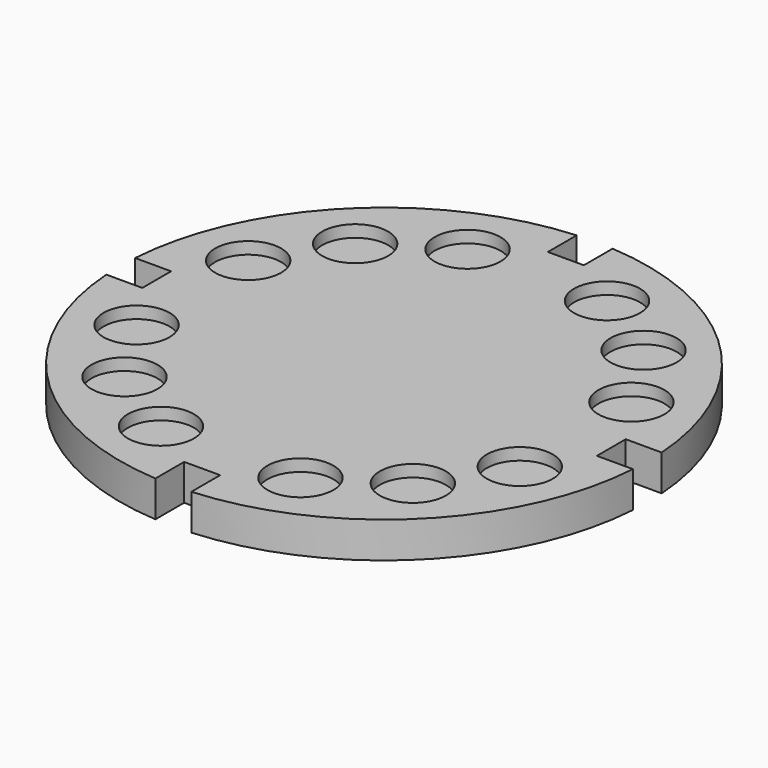
from build123d import *

# Parameters (mm, degrees)
F0_R            = 17.4625
F0_W            = 19.05
F0_H            = 6.35
F1_DEPTH        = 19.05
F2_DEPTH        = 6.35
F2_COPIES_COUNT = 4
F3_DEPTH        = 19.051
F3_COPIES_COUNT = 4


# Not quite as in the source:
# - a pattern or mirror of a feature is missing from the dataset's text; its kind, count and spacing are read off the source's solid


with BuildPart() as f1:
    # F0 (on Top) → F1 (new body)
    with BuildSketch(Plane.XY):
        with BuildLine():
            ThreePointArc((-9.525, 139.3749058296), (-95.3557746023, -102.0948884617), (139.7, 0))
            ThreePointArc((139.7, 0), (102.0948884617, 95.3557746023), (9.525, 139.3749058296))
            Line((9.525, 139.3749058296), (9.525, 120.3249058296))
            Line((9.525, 120.3249058296), (9.525, 113.9749058296))
            Line((9.525, 113.9749058296), (-9.525, 113.9749058296))
            Line((-9.525, 113.9749058296), (-9.525, 120.3249058296))
            Line((-9.525, 120.3249058296), (-9.525, 139.3749058296))
        make_face()
        with Locations((101.4398184138, 36.921074472)):
            Circle(F0_R, mode=Mode.SUBTRACT)
        with Locations((36.921074472, 101.4398184138)):
            Circle(F0_R, mode=Mode.SUBTRACT)
        with Locations((76.3321770291, 76.3321770291)):
            Circle(F0_R, mode=Mode.SUBTRACT)
        with BuildLine():
            Line((9.525, 120.3249058296), (9.525, 139.3749058296))
            ThreePointArc((9.525, 139.3749058296), (0, 139.7), (-9.525, 139.3749058296))
            Line((-9.525, 139.3749058296), (-9.525, 120.3249058296))
            Line((-9.525, 120.3249058296), (9.525, 120.3249058296))
        make_face()
        with Locations((36.921074472, 101.4398184138)):
            Circle(F0_R)
        with Locations((76.3321770291, 76.3321770291)):
            Circle(F0_R)
        with Locations((101.4398184138, 36.921074472)):
            Circle(F0_R)
        with Locations((0, 117.1499058296)):
            Rectangle(F0_W, F0_H)
    extrude(amount=-F1_DEPTH)

    # F0 (on Top) → F2 (cut)
    with BuildSketch(Plane.XY):
        with Locations((36.921074472, 101.4398184138)):
            Circle(F0_R)
        with Locations((76.3321770291, 76.3321770291)):
            Circle(F0_R)
        with Locations((101.4398184138, 36.921074472)):
            Circle(F0_R)
    f2 = extrude(amount=-F2_DEPTH, mode=Mode.SUBTRACT)

    # F2_copies: F2 ×4 about axis
    f2_copies_axis = Axis((0, 0, 0), (0, 0, 1))
    for i in range(1, F2_COPIES_COUNT):
        add(f2.rotate(f2_copies_axis, i * 360 / F2_COPIES_COUNT), mode=Mode.SUBTRACT)

    # F0 (on Top) → F3 (cut, through all)
    with BuildSketch(Plane.XY):
        with BuildLine():
            Line((9.525, 120.3249058296), (9.525, 139.3749058296))
            ThreePointArc((9.525, 139.3749058296), (0, 139.7), (-9.525, 139.3749058296))
            Line((-9.525, 139.3749058296), (-9.525, 120.3249058296))
            Line((-9.525, 120.3249058296), (9.525, 120.3249058296))
        make_face()
    f3 = extrude(amount=-F3_DEPTH, mode=Mode.SUBTRACT)

    # F3_copies: F3 ×4 about axis
    f3_copies_axis = Axis((0, 0, 0), (0, 0, 1))
    for i in range(1, F3_COPIES_COUNT):
        add(f3.rotate(f3_copies_axis, i * 360 / F3_COPIES_COUNT), mode=Mode.SUBTRACT)


solid = f1.part
